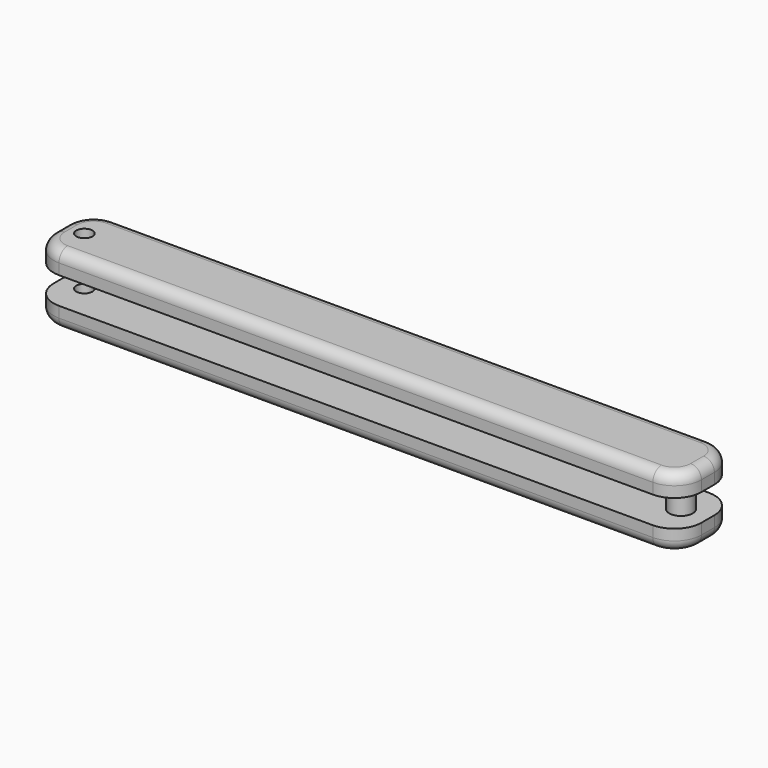
from build123d import *

# Parameters (mm, degrees)
F0_W          = 120
F0_H          = 13
F0_R          = 1.5
F1_DEPTH      = 13
F2_W          = 120
F2_H          = 5
F3_DEPTH      = 8
F3_DEPTH_BACK = 8
F4_R          = 2.1741492727
F5_DEPTH      = 13
F6_R          = 2
F7_T1_DEPTH   = 16.5
F7_T3_DEPTH   = 16.5
F7_T6_ANGLE   = 90
F7_T8_ANGLE   = 90
F7_T10_ANGLE  = 90
F7_T12_ANGLE  = 90
F7_T14_ANGLE  = 90
F7_T16_ANGLE  = 90
F7_T18_ANGLE  = 90
F7_T20_ANGLE  = 90


# Not quite as in the source:
# - a fillet or chamfer that OpenCascade refuses, or shapes differently, is made with other operations: its cross-section is extruded or revolved along the edge and cut away or added


with BuildPart() as f1:
    # F0 (on Top) → F1 (new body)
    with BuildSketch(Plane.XY):
        Rectangle(F0_W, F0_H)
        with Locations((-55.5, 0)):
            Circle(F0_R, mode=Mode.SUBTRACT)
    extrude(amount=F1_DEPTH)

    # F2 (on Front) → F3 (cut, two sides)
    with BuildSketch(Plane.XZ) as f3_sk:
        with Locations((0, 6.5)):
            Rectangle(F2_W, F2_H)
    extrude(amount=-F3_DEPTH, mode=Mode.SUBTRACT)
    extrude(f3_sk.sketch, amount=F3_DEPTH_BACK, mode=Mode.SUBTRACT)

    # F4 (on Top) → F5 (join)
    with BuildSketch(Plane.XY):
        with Locations((55.0134144723, 0)):
            Circle(F4_R)
    extrude(amount=F5_DEPTH)

    # F6
    f6_edges = [f1.edges().sort_by_distance(p)[0] for p in [
        (0, -6.5, 13),
        (-60, 0, 13),
        (0, 6.5, 13),
        (60, 0, 13),
        (-60, 0, 0),
        (0, -6.5, 0),
        (60, 0, 0),
        (0, 6.5, 0),
    ]]
    fillet(f6_edges, radius=F6_R)

    # F7: fillet of radius 5 on 8 edges, made by hand

    # F7_s2 → F7_t1 (cut)
    with BuildSketch(Plane.XY.offset(-3.5)):
        with BuildLine():
            ThreePointArc((-55, -6.5), (-58.5355339059, -5.0355339059), (-60, -1.5))
            Line((-60, -1.5), (-60, -6.5))
            Line((-60, -6.5), (-55, -6.5))
        make_face()
        with BuildLine():
            ThreePointArc((-55, 6.5), (-58.5355339059, 5.0355339059), (-60, 1.5))
            Line((-60, 1.5), (-60, 6.5))
            Line((-60, 6.5), (-55, 6.5))
        make_face()
        with BuildLine():
            ThreePointArc((60, -1.5), (58.5355339059, -5.0355339059), (55, -6.5))
            Line((55, -6.5), (60, -6.5))
            Line((60, -6.5), (60, -1.5))
        make_face()
        with BuildLine():
            ThreePointArc((60, 1.5), (58.5355339059, 5.0355339059), (55, 6.5))
            Line((55, 6.5), (60, 6.5))
            Line((60, 6.5), (60, 1.5))
        make_face()
    extrude(amount=F7_T1_DEPTH, mode=Mode.SUBTRACT)

    # F7_s4 → F7_t3 (cut)
    with BuildSketch(Plane.XY):
        with BuildLine():
            ThreePointArc((-55, -6.5), (-58.5355339059, -5.0355339059), (-60, -1.5))
            Line((-60, -1.5), (-60, -6.5))
            Line((-60, -6.5), (-55, -6.5))
        make_face()
        with BuildLine():
            ThreePointArc((-55, 6.5), (-58.5355339059, 5.0355339059), (-60, 1.5))
            Line((-60, 1.5), (-60, 6.5))
            Line((-60, 6.5), (-55, 6.5))
        make_face()
        with BuildLine():
            ThreePointArc((60, -1.5), (58.5355339059, -5.0355339059), (55, -6.5))
            Line((55, -6.5), (60, -6.5))
            Line((60, -6.5), (60, -1.5))
        make_face()
        with BuildLine():
            ThreePointArc((60, 1.5), (58.5355339059, 5.0355339059), (55, 6.5))
            Line((55, 6.5), (60, 6.5))
            Line((60, 6.5), (60, 1.5))
        make_face()
    extrude(amount=F7_T3_DEPTH, mode=Mode.SUBTRACT)

    # F7_s5 → F7_t6 (revolve, cut)
    with BuildSketch(Plane.YZ.offset(55)):
        with BuildLine():
            ThreePointArc((4.5, 0), (5.9142135624, 0.5857864376), (6.5, 2))
            Line((6.5, 2), (6.5, 0))
            Line((6.5, 0), (4.5, 0))
        make_face()
    revolve(axis=Axis((55, 1.5, 0), (0, 0, -1)), revolution_arc=F7_T6_ANGLE, mode=Mode.SUBTRACT)

    # F7_s7 → F7_t8 (revolve, cut)
    with BuildSketch(Plane.XZ.offset(1.5)):
        with BuildLine():
            ThreePointArc((58, 0), (59.4142135624, 0.5857864376), (60, 2))
            Line((60, 2), (60, 0))
            Line((60, 0), (58, 0))
        make_face()
    revolve(axis=Axis((55, -1.5, 0), (0, 0, -1)), revolution_arc=F7_T8_ANGLE, mode=Mode.SUBTRACT)

    # F7_s9 → F7_t10 (revolve, cut)
    with BuildSketch(Plane.XZ.offset(-1.5)):
        with BuildLine():
            ThreePointArc((58, 13), (59.4142135624, 12.4142135624), (60, 11))
            Line((60, 11), (60, 13))
            Line((60, 13), (58, 13))
        make_face()
    revolve(axis=Axis((55, 1.5, 13), (0, 0, 1)), revolution_arc=F7_T10_ANGLE, mode=Mode.SUBTRACT)

    # F7_s11 → F7_t12 (revolve, cut)
    with BuildSketch(Plane.YZ.offset(55)):
        with BuildLine():
            ThreePointArc((-4.5, 13), (-5.9142135624, 12.4142135624), (-6.5, 11))
            Line((-6.5, 11), (-6.5, 13))
            Line((-6.5, 13), (-4.5, 13))
        make_face()
    revolve(axis=Axis((55, -1.5, 13), (0, 0, 1)), revolution_arc=F7_T12_ANGLE, mode=Mode.SUBTRACT)

    # F7_s13 → F7_t14 (revolve, cut)
    with BuildSketch(Plane.XZ.offset(-1.5)):
        with BuildLine():
            ThreePointArc((-58, 0), (-59.4142135624, 0.5857864376), (-60, 2))
            Line((-60, 2), (-60, 0))
            Line((-60, 0), (-58, 0))
        make_face()
    revolve(axis=Axis((-55, 1.5, 0), (0, 0, -1)), revolution_arc=F7_T14_ANGLE, mode=Mode.SUBTRACT)

    # F7_s15 → F7_t16 (revolve, cut)
    with BuildSketch(Plane.YZ.offset(-55)):
        with BuildLine():
            ThreePointArc((-4.5, 0), (-5.9142135624, 0.5857864376), (-6.5, 2))
            Line((-6.5, 2), (-6.5, 0))
            Line((-6.5, 0), (-4.5, 0))
        make_face()
    revolve(axis=Axis((-55, -1.5, 0), (0, 0, -1)), revolution_arc=F7_T16_ANGLE, mode=Mode.SUBTRACT)

    # F7_s17 → F7_t18 (revolve, cut)
    with BuildSketch(Plane.YZ.offset(-55)):
        with BuildLine():
            ThreePointArc((4.5, 13), (5.9142135624, 12.4142135624), (6.5, 11))
            Line((6.5, 11), (6.5, 13))
            Line((6.5, 13), (4.5, 13))
        make_face()
    revolve(axis=Axis((-55, 1.5, 13), (0, 0, 1)), revolution_arc=F7_T18_ANGLE, mode=Mode.SUBTRACT)

    # F7_s19 → F7_t20 (revolve, cut)
    with BuildSketch(Plane.XZ.offset(1.5)):
        with BuildLine():
            ThreePointArc((-58, 13), (-59.4142135624, 12.4142135624), (-60, 11))
            Line((-60, 11), (-60, 13))
            Line((-60, 13), (-58, 13))
        make_face()
    revolve(axis=Axis((-55, -1.5, 13), (0, 0, 1)), revolution_arc=F7_T20_ANGLE, mode=Mode.SUBTRACT)


solid = f1.part
